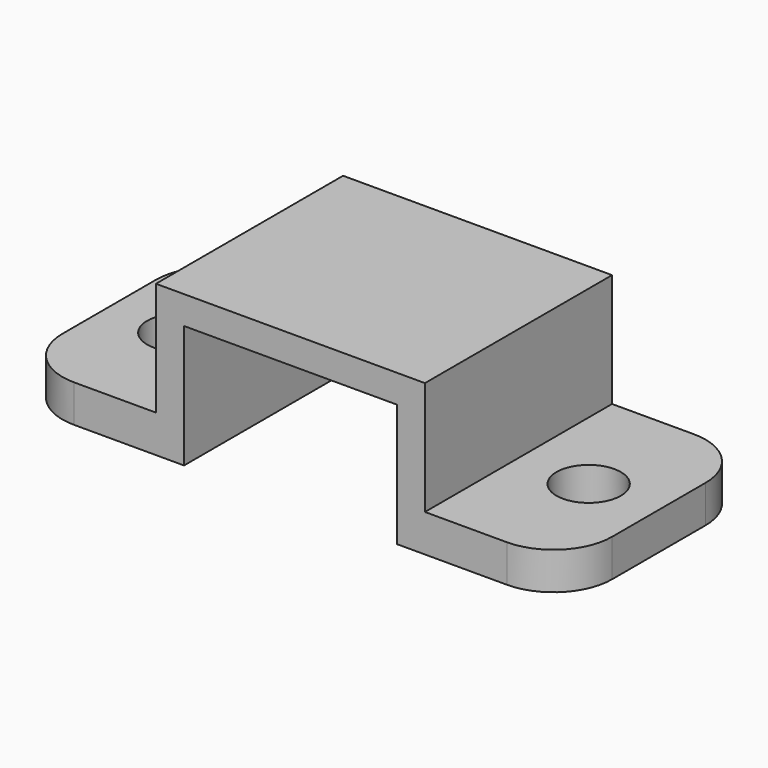
from build123d import *

# Parameters (mm, degrees)
F0_W         = 12
F0_H         = 3.2
F1_DEPTH     = 20
F3_D         = 5.5
F4_W         = 18.2
F4_H         = 1.6
F5_DEPTH     = 0.9
F6_T1_DEPTH  = 18.2
F6_T6_DEPTH  = 18.2
F6_T11_DEPTH = 18.2
F6_T16_DEPTH = 18.2
F6_T21_DEPTH = 18.2
F6_T26_DEPTH = 18.2
F6_T31_DEPTH = 18.2
F6_T36_DEPTH = 18.2
F7_R         = 5


# Not quite as in the source:
# - a fillet or chamfer that OpenCascade refuses, or shapes differently, is made with other operations: its cross-section is extruded or revolved along the edge and cut away or added


with BuildPart() as f1:
    # F0 (on Front) → F1 (new body)
    with BuildSketch(Plane.XZ):
        Polygon((-9.1, 10.5), (0, 10.5), (0, 12.9), (-11.5, 12.9), (-11.5, 3.2), (-11.5, 0), (-9.1, 0), align=None)
        with Locations((-17.5, 1.6)):
            Rectangle(F0_W, F0_H)
        Polygon((0, 12.9), (0, 10.5), (9.1, 10.5), (9.1, 0), (11.5, 0), (11.5, 3.2), (11.5, 12.9), align=None)
        with Locations((17.5, 1.6)):
            Rectangle(F0_W, F0_H)
    extrude(amount=F1_DEPTH)

    # F3 (through all)
    with Locations(Plane.XY.offset(3.2)):
        with Locations((-17.5, -10), (17.5, -10)):
            Hole(F3_D / 2)

    # F4 (on face) → F5 (join)
    with BuildSketch(Plane(origin=(0, 0, 10.5), x_dir=(1, 0, 0), z_dir=(0, 0, -1))):
        with Locations((0, 0.8)):
            Rectangle(F4_W, F4_H)
        with Locations((0, 4)):
            Rectangle(F4_W, F4_H)
        with Locations((0, 7.2)):
            Rectangle(F4_W, F4_H)
        with Locations((0, 10.4)):
            Rectangle(F4_W, F4_H)
    extrude(amount=F5_DEPTH)

    # F6: chamfer of 1 on 8 edges, made by hand

    # F6_s2 → F6_t1 (cut)
    with BuildSketch(Plane.YZ.offset(-9.1)):
        Polygon((-1, 9.6), (0, 10.6), (0, 9.6), align=None)
    extrude(amount=F6_T1_DEPTH, mode=Mode.SUBTRACT)


with BuildPart() as f6_tool4:
    # F6_s5 → F6_t6 (new body)
    with BuildSketch(Plane.YZ.offset(9.1)):
        Polygon((-1.6, 10.6), (-0.6, 9.6), (-1.6, 9.6), align=None)
    extrude(amount=-F6_T6_DEPTH)

    split(bisect_by=Plane.XY.offset(10.5), keep=Keep.BOTTOM)


with BuildPart() as f1_1:
    add(f1.part)

    # F6_t3: cut F6_tool4
    add(f6_tool4.part, mode=Mode.SUBTRACT)


with BuildPart() as f6_tool9:
    # F6_s10 → F6_t11 (new body)
    with BuildSketch(Plane.YZ.offset(-9.1)):
        Polygon((-3.2, 10.6), (-4.2, 9.6), (-3.2, 9.6), align=None)
    extrude(amount=F6_T11_DEPTH)

    split(bisect_by=Plane.XY.offset(10.5), keep=Keep.BOTTOM)


with BuildPart() as f1_2:
    add(f1_1.part)

    # F6_t8: cut F6_tool9
    add(f6_tool9.part, mode=Mode.SUBTRACT)


with BuildPart() as f6_tool14:
    # F6_s15 → F6_t16 (new body)
    with BuildSketch(Plane.YZ.offset(9.1)):
        Polygon((-4.8, 10.6), (-3.8, 9.6), (-4.8, 9.6), align=None)
    extrude(amount=-F6_T16_DEPTH)

    split(bisect_by=Plane.XY.offset(10.5), keep=Keep.BOTTOM)


with BuildPart() as f1_3:
    add(f1_2.part)

    # F6_t13: cut F6_tool14
    add(f6_tool14.part, mode=Mode.SUBTRACT)


with BuildPart() as f6_tool19:
    # F6_s20 → F6_t21 (new body)
    with BuildSketch(Plane.YZ.offset(-9.1)):
        Polygon((-7.4, 9.6), (-6.4, 10.6), (-6.4, 9.6), align=None)
    extrude(amount=F6_T21_DEPTH)

    split(bisect_by=Plane.XY.offset(10.5), keep=Keep.BOTTOM)


with BuildPart() as f1_4:
    add(f1_3.part)

    # F6_t18: cut F6_tool19
    add(f6_tool19.part, mode=Mode.SUBTRACT)


with BuildPart() as f6_tool24:
    # F6_s25 → F6_t26 (new body)
    with BuildSketch(Plane.YZ.offset(9.1)):
        Polygon((-8, 10.6), (-7, 9.6), (-8, 9.6), align=None)
    extrude(amount=-F6_T26_DEPTH)

    split(bisect_by=Plane.XY.offset(10.5), keep=Keep.BOTTOM)


with BuildPart() as f1_5:
    add(f1_4.part)

    # F6_t23: cut F6_tool24
    add(f6_tool24.part, mode=Mode.SUBTRACT)


with BuildPart() as f6_tool29:
    # F6_s30 → F6_t31 (new body)
    with BuildSketch(Plane.YZ.offset(-9.1)):
        Polygon((-10.6, 9.6), (-9.6, 10.6), (-9.6, 9.6), align=None)
    extrude(amount=F6_T31_DEPTH)

    split(bisect_by=Plane.XY.offset(10.5), keep=Keep.BOTTOM)


with BuildPart() as f1_6:
    add(f1_5.part)

    # F6_t28: cut F6_tool29
    add(f6_tool29.part, mode=Mode.SUBTRACT)


with BuildPart() as f6_tool34:
    # F6_s35 → F6_t36 (new body)
    with BuildSketch(Plane.YZ.offset(9.1)):
        Polygon((-11.2, 10.6), (-10.2, 9.6), (-11.2, 9.6), align=None)
    extrude(amount=-F6_T36_DEPTH)

    split(bisect_by=Plane.XY.offset(10.5), keep=Keep.BOTTOM)


with BuildPart() as f1_7:
    add(f1_6.part)

    # F6_t33: cut F6_tool34
    add(f6_tool34.part, mode=Mode.SUBTRACT)

    # F7
    f7_edges = [f1_7.edges().sort_by_distance(p)[0] for p in [
        (-23.5, -20, 1.6),
        (23.5, -20, 1.6),
        (23.5, 0, 1.6),
        (-23.5, 0, 1.6),
    ]]
    fillet(f7_edges, radius=F7_R)


solid = f1_7.part
